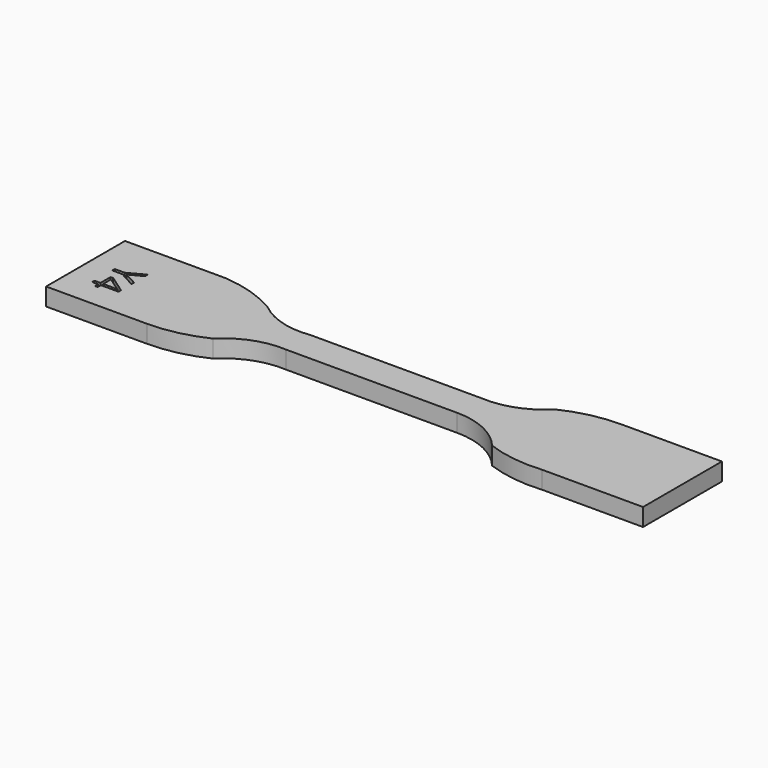
from build123d import *

# Parameters (mm, degrees)
F1_DEPTH     = 3.4
F2_TEXT_SIZE = 7.0564552314
F3_DEPTH     = 1


# Not quite as in the source:
# - Text() gives the source's letters only with a copy of the font that has no kerning and outlines rounded to 1/6400 em; it was checked with that copy


with BuildPart() as f1:
    # F0 (on Top) → F1 (new body)
    with BuildSketch(Plane.XY):
        with BuildLine():
            Line((-14.4320548165, 19.7811394548), (-33.8720548165, 19.7811394548))
            Line((-33.8720548165, 19.7811394548), (-33.8720548165, 0.7811394548))
            Line((-33.8720548165, 0.7811394548), (-14.4320548165, 0.7811394548))
            ThreePointArc((-14.4320548165, 0.7811394548), (-8.9053122052, 1.3996892086), (-3.6520548165, 3.2247301661))
            ThreePointArc((-3.6520548165, 3.2247301661), (1.3014698263, 6.4128780055), (7.1279451835, 7.2811394548))
            Line((7.1279451835, 7.2811394548), (40.1279451835, 7.2811394548))
            ThreePointArc((40.1279451835, 7.2811394548), (46.0837574042, 5.9511158081), (50.9079451835, 2.2137538538))
            ThreePointArc((50.9079451835, 2.2137538538), (56.2191047011, 0.9041953221), (61.6879451835, 0.7811394548))
            Line((61.6879451835, 0.7811394548), (81.1279451835, 0.7811394548))
            Line((81.1279451835, 0.7811394548), (81.1279451835, 19.7811394548))
            Line((81.1279451835, 19.7811394548), (61.6879451835, 19.7811394548))
            ThreePointArc((61.6879451835, 19.7811394548), (56.1612025723, 19.162589701), (50.9079451835, 17.3375487435))
            ThreePointArc((50.9079451835, 17.3375487435), (45.9544205407, 14.1494009041), (40.1279451835, 13.2811394548))
            Line((40.1279451835, 13.2811394548), (7.1279451835, 13.2811394548))
            ThreePointArc((7.1279451835, 13.2811394548), (1.4167452884, 13.6925537245), (-3.6520548165, 16.3560723447))
            ThreePointArc((-3.6520548165, 16.3560723447), (-8.8458057958, 18.686276846), (-14.4320548165, 19.7811394548))
        make_face()
    extrude(amount=F1_DEPTH)

    # F2 (on face) → F3 (cut)
    with BuildSketch(Plane.XY.offset(3.4)):
        with Locations(Location((-29.3720550835, 13.353464842), (0, 0, -90))):
            Text('Y4', F2_TEXT_SIZE, font='Open Sans', text_align=(TextAlign.LEFT, TextAlign.BOTTOM))
    extrude(amount=-F3_DEPTH, mode=Mode.SUBTRACT)


solid = f1.part
